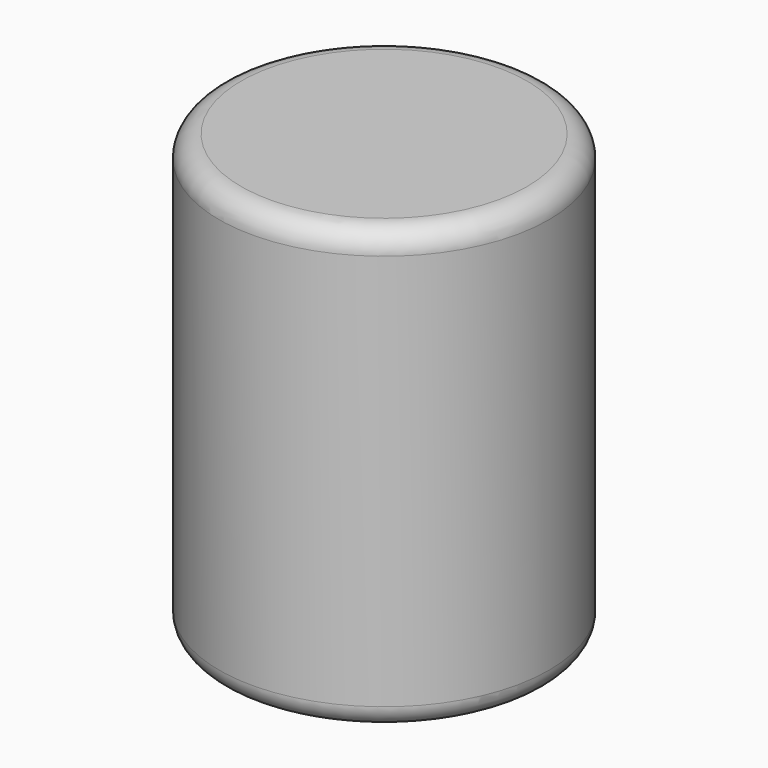
from build123d import *

# Parameters (mm, degrees)
F0_R     = 38.1
F1_DEPTH = 101.6
F2_R     = 34.29
F3_DEPTH = 95.25


# Not quite as in the source:
# - a fillet or chamfer that OpenCascade refuses, or shapes differently, is made with other operations: its cross-section is extruded or revolved along the edge and cut away or added


with BuildPart() as f1:
    # F0 (on Top) → F1 (new body)
    with BuildSketch(Plane.XY):
        Circle(F0_R)
    extrude(amount=F1_DEPTH)

    # F2 (on Top) → F3 (cut)
    with BuildSketch(Plane.XY):
        Circle(F2_R)
    extrude(amount=F3_DEPTH, mode=Mode.SUBTRACT)

    # F4: fillet of radius 5.08 on 2 edges, made by hand

    # F4_s1 → F4_t2 (revolve, cut)
    with BuildSketch(Plane.XZ):
        with BuildLine():
            ThreePointArc((38.1, 4.9186888497), (37.0360926284, 1.8078368763), (34.29, 0))
            Line((34.29, 0), (38.1, 0))
            Line((38.1, 0), (38.1, 4.9186888497))
        make_face()
    revolve(axis=Axis((0, 0, 0), (0, 0, 1)), mode=Mode.SUBTRACT)

    # F4_s3 → F4_t4 (revolve, cut)
    with BuildSketch(Plane.XZ):
        with BuildLine():
            ThreePointArc((38.1, 96.52), (36.6121024484, 100.1121024484), (33.02, 101.6))
            Line((33.02, 101.6), (38.1, 101.6))
            Line((38.1, 101.6), (38.1, 96.52))
        make_face()
    revolve(axis=Axis((0, 0, 101.6), (0, 0, 1)), mode=Mode.SUBTRACT)


solid = f1.part
